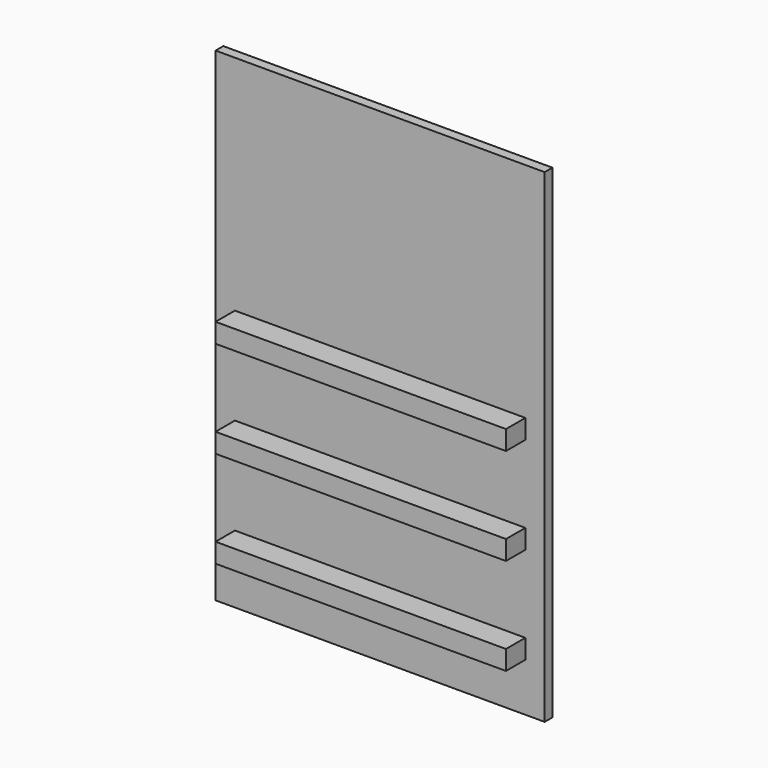
from build123d import *

# Parameters (mm, degrees)
F0_W     = 340
F0_H     = 500
F0_W_2   = 300
F0_H_2   = 20
F1_DEPTH = 10
F2_DEPTH = 35


# Not quite as in the source:
# - a feature names something its author has since deleted; it is built from what else it names


with BuildPart() as f1:
    # F0 (on Front) → F1 (new body)
    with BuildSketch(Plane.XZ):
        with Locations((-54.2285538465, 60.7086803179)):
            Rectangle(F0_W, F0_H)
        with Locations((-54.2285538465, -129.2913196821)):
            Rectangle(F0_W_2, F0_H_2, mode=Mode.SUBTRACT)
        with Locations((-54.2285538465, -29.2913196821)):
            Rectangle(F0_W_2, F0_H_2, mode=Mode.SUBTRACT)
        with Locations((-54.2285538465, 70.7086803179)):
            Rectangle(F0_W_2, F0_H_2, mode=Mode.SUBTRACT)
    extrude(amount=F1_DEPTH)

    # F0 (on Front) → F2 (join)
    with BuildSketch(Plane.XZ):
        with Locations((-54.2285538465, 70.7086803179)):
            Rectangle(F0_W_2, F0_H_2)
        with Locations((-54.2285538465, -29.2913196821)):
            Rectangle(F0_W_2, F0_H_2)
        with Locations((-54.2285538465, -129.2913196821)):
            Rectangle(F0_W_2, F0_H_2)
    extrude(amount=F2_DEPTH)


solid = f1.part
